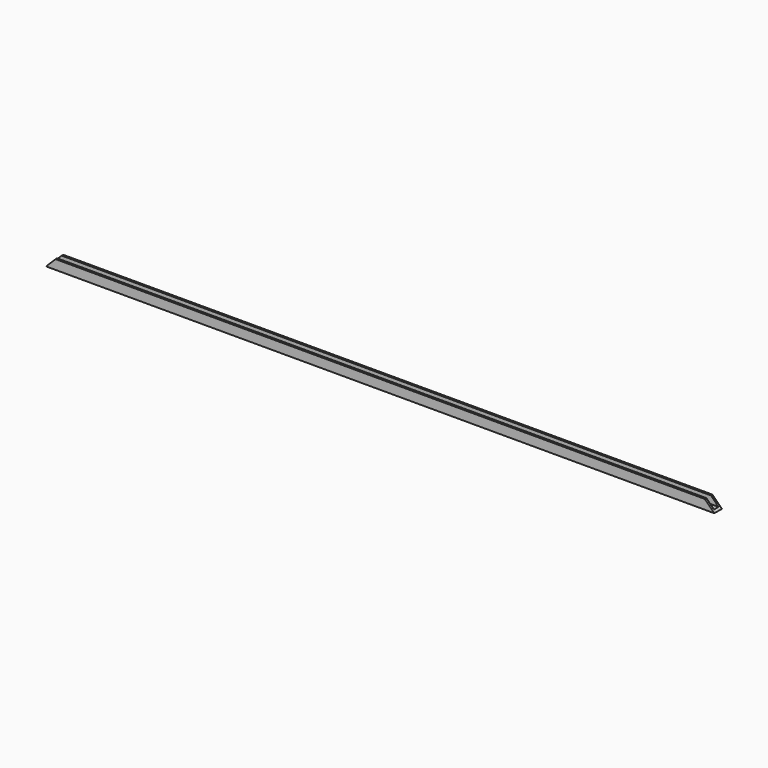
from build123d import *

# Parameters (mm, degrees)
F1_DEPTH   = 704
F2_C1_SIZE = 9.9999
F2_C2_SIZE = 9.9999


# Not quite as in the source:
# - a fillet or chamfer is up to 0.001 mm smaller than in the source, because OpenCascade refuses the exact size


with BuildPart() as f1:
    # F0 (on Right) → F1 (new body)
    with BuildSketch(Plane.YZ):
        Polygon((-3, 5), (-5, 5), (-5, -5), (5, -5), (5, 5), (3, 5), (3, -3), (-3, -3), align=None)
    extrude(amount=F1_DEPTH)

    # F2: chamfer of 10 on 3 edges, made by hand

    # F2_c1 (size 10 in the source; OpenCascade refuses exactly that, so slightly less here)
    f2_c1_edges = [f1.edges().sort_by_distance(p)[0] for p in [
        (0, -4, 5),
    ]]
    chamfer(f2_c1_edges, length=F2_C1_SIZE)

    # F2_c2 (size 10 in the source; OpenCascade refuses exactly that, so slightly less here)
    f2_c2_edges = [f1.edges().sort_by_distance(p)[0] for p in [
        (704, -4, 5),
    ]]
    chamfer(f2_c2_edges, length=F2_C2_SIZE)


solid = f1.part
